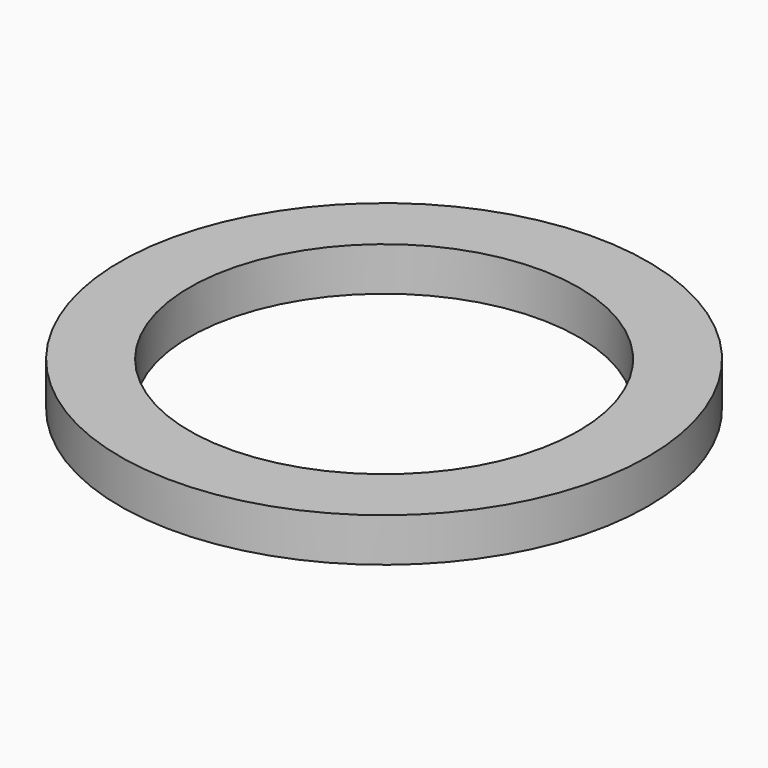
from build123d import *

# Parameters (mm, degrees)
F0_R     = 71.6667428664
F0_R_2   = 52.8042523371
F1_DEPTH = 11.8537191302


# Not quite as in the source:
# - the program builds the solid bodies; features that only make, move or delete a surface that nothing else refers to are left out


with BuildPart() as f1:
    # F0 (on Top) → F1 (new body)
    with BuildSketch(Plane.XY):
        Circle(F0_R)
        Circle(F0_R_2, mode=Mode.SUBTRACT)
    extrude(amount=F1_DEPTH)


solid = f1.part
